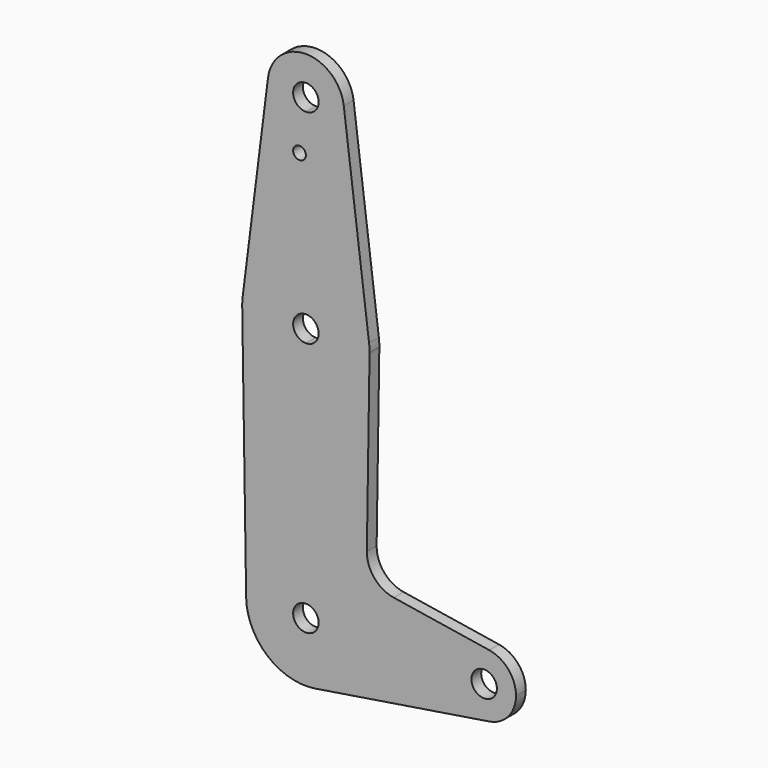
from build123d import *

# Parameters (mm, degrees)
F0_R     = 1.5875
F1_DEPTH = 3.048


# Not quite as in the source:
# - a feature names something its author has since deleted; it is built from what else it names


with BuildPart() as f1:
    # F0 (on Front) → F1 (new body)
    with BuildSketch(Plane.XZ):
        with BuildLine():
            Line((0, 3.0934604908), (0, 0))
            Line((0, 0), (0, -9.6065395092))
            ThreePointArc((0, -9.6065395092), (11.1386616751, -5.0428542466), (15.8731222627, 6.024299409))
            ThreePointArc((15.8731222627, 6.024299409), (15.8745305587, 6.1463763397), (15.875, 6.2684604908))
            ThreePointArc((15.875, 6.2684604908), (15.8438414904, 7.2625992274), (15.7504882737, 8.2528354908))
            ThreePointArc((15.7504882737, 8.2528354908), (10.5003255158, 18.1747104908), (0, 22.1434604908))
            Line((0, 22.1434604908), (0, 9.4434604908))
            ThreePointArc((0, 9.4434604908), (2.2450640303, 8.513524521), (3.175, 6.2684604908))
            ThreePointArc((3.175, 6.2684604908), (2.2450640303, 4.0233964605), (0, 3.0934604908))
        make_face()
        with BuildLine():
            Line((0, -9.6065395092), (0, 0))
            Line((0, 0), (0, 3.0934604908))
            ThreePointArc((0, 3.0934604908), (-3.175, 6.2684604908), (0, 9.4434604908))
            Line((0, 9.4434604908), (0, 22.1434604908))
            ThreePointArc((0, 22.1434604908), (-10.5003255158, 18.1747104908), (-15.7504882737, 8.2528354908))
            ThreePointArc((-15.7504882737, 8.2528354908), (-15.8510182356, 7.1407252981), (-15.8731222627, 6.024299409))
            ThreePointArc((-15.8731222627, 6.024299409), (-11.1386616751, -5.0428542466), (0, -9.6065395092))
        make_face()
        with BuildLine():
            ThreePointArc((15.8731222627, 6.024299409), (11.1386616751, -5.0428542466), (0, -9.6065395092))
            Line((0, -9.6065395092), (0, -42.3331838364))
            ThreePointArc((0, -42.3331838364), (10.5347283248, -46.6968111845), (14.8983556728, -57.2315395092))
            Line((14.8983556728, -57.2315395092), (36.5125, -57.2315395092))
            ThreePointArc((36.5125, -57.2315395092), (39.2955109449, -51.1953860295), (45.6930099416, -49.3919711196))
            Line((45.6930099416, -49.3919711196), (21.9056452954, -45.6203437456))
            ThreePointArc((21.9056452954, -45.6203437456), (17.0653083108, -42.8843212703), (15.2013844237, -37.6459561768))
            Line((15.2013844237, -37.6459561768), (15.8731222627, 6.024299409))
        make_face()
        with BuildLine():
            Line((0, -42.3331838364), (0, -9.6065395092))
            ThreePointArc((0, -9.6065395092), (-11.1386616751, -5.0428542466), (-15.8731222627, 6.024299409))
            Line((-15.8731222627, 6.024299409), (-14.8965934556, -57.4606795809))
            ThreePointArc((-14.8965934556, -57.4606795809), (-10.6154324462, -46.778138353), (0, -42.3331838364))
        make_face()
        with BuildLine():
            ThreePointArc((14.8983556728, -57.2315395092), (10.5347283248, -46.6968111845), (0, -42.3331838364))
            Line((0, -42.3331838364), (0, -54.0565395092))
            ThreePointArc((0, -54.0565395092), (2.2450640303, -54.986475479), (3.175, -57.2315395092))
            Line((3.175, -57.2315395092), (14.8983556728, -57.2315395092))
        make_face()
        with BuildLine():
            Line((0, -54.0565395092), (0, -42.3331838364))
            ThreePointArc((0, -42.3331838364), (-10.6154324462, -46.778138353), (-14.8965934556, -57.4606795809))
            ThreePointArc((-14.8965934556, -57.4606795809), (-9.5873458416, -68.6352144199), (2.3330776963, -71.9460816433))
            ThreePointArc((2.3330776963, -71.9460816433), (11.32960774, -66.9062999823), (14.8983556728, -57.2315395092))
            Line((14.8983556728, -57.2315395092), (3.175, -57.2315395092))
            ThreePointArc((3.175, -57.2315395092), (-2.2450640303, -59.4766035395), (0, -54.0565395092))
        make_face()
        with BuildLine():
            Line((36.5125, -57.2315395092), (14.8983556728, -57.2315395092))
            ThreePointArc((14.8983556728, -57.2315395092), (11.32960774, -66.9062999823), (2.3330776963, -71.9460816433))
            Line((2.3330776963, -71.9460816433), (45.6930099416, -65.0711078988))
            ThreePointArc((45.6930099416, -65.0711078988), (39.2955109449, -63.2676929889), (36.5125, -57.2315395092))
        make_face()
        with BuildLine():
            Line((-9.4502929642, 58.2590854908), (-15.7504882737, 8.2528354908))
            ThreePointArc((-15.7504882737, 8.2528354908), (-10.5003255158, 18.1747104908), (0, 22.1434604908))
            Line((0, 22.1434604908), (0, 44.3480842421))
            Line((0, 44.3480842421), (0, 47.5434604908))
            ThreePointArc((0, 47.5434604908), (-7.14375, 50.7682651813), (-9.4502929642, 58.2590854908))
        make_face()
        with Locations((-1.5875, 44.3480842421)):
            Circle(F0_R, mode=Mode.SUBTRACT)
        with BuildLine():
            Line((0, 44.3480842421), (0, 22.1434604908))
            ThreePointArc((0, 22.1434604908), (10.5003255158, 18.1747104908), (15.7504882737, 8.2528354908))
            Line((15.7504882737, 8.2528354908), (9.4502929642, 58.2590854908))
            ThreePointArc((9.4502929642, 58.2590854908), (9.5063048942, 57.6649437327), (9.525, 57.0684604908))
            ThreePointArc((9.525, 57.0684604908), (6.7351920908, 50.3332684), (0, 47.5434604908))
            Line((0, 47.5434604908), (0, 44.3480842421))
        make_face()
        with BuildLine():
            ThreePointArc((45.6930099416, -49.3919711196), (39.2955109449, -51.1953860295), (36.5125, -57.2315395092))
            ThreePointArc((36.5125, -57.2315395092), (39.2955109449, -63.2676929889), (45.6930099416, -65.0711078988))
            ThreePointArc((45.6930099416, -65.0711078988), (50.4861534797, -62.3860285644), (52.3875, -57.2315395092))
            ThreePointArc((52.3875, -57.2315395092), (50.4861534797, -52.0770504541), (45.6930099416, -49.3919711196))
        make_face()
        with BuildLine():
            ThreePointArc((47.625, -57.2315395092), (44.45, -60.4065395092), (41.275, -57.2315395092))
            ThreePointArc((41.275, -57.2315395092), (44.45, -54.0565395092), (47.625, -57.2315395092))
        make_face(mode=Mode.SUBTRACT)
        with BuildLine():
            ThreePointArc((9.4502929642, 58.2590854908), (0, 66.5934604908), (-9.4502929642, 58.2590854908))
            ThreePointArc((-9.4502929642, 58.2590854908), (-7.14375, 50.7682651813), (0, 47.5434604908))
            ThreePointArc((0, 47.5434604908), (6.7351920908, 50.3332684), (9.525, 57.0684604908))
            ThreePointArc((9.525, 57.0684604908), (9.5063048942, 57.6649437327), (9.4502929642, 58.2590854908))
        make_face()
        with BuildLine():
            ThreePointArc((3.175, 57.0684604908), (2.2450640303, 54.8233964605), (0, 53.8934604908))
            ThreePointArc((0, 53.8934604908), (-2.2450640303, 59.313524521), (3.175, 57.0684604908))
        make_face(mode=Mode.SUBTRACT)
    extrude(amount=F1_DEPTH)


solid = f1.part
